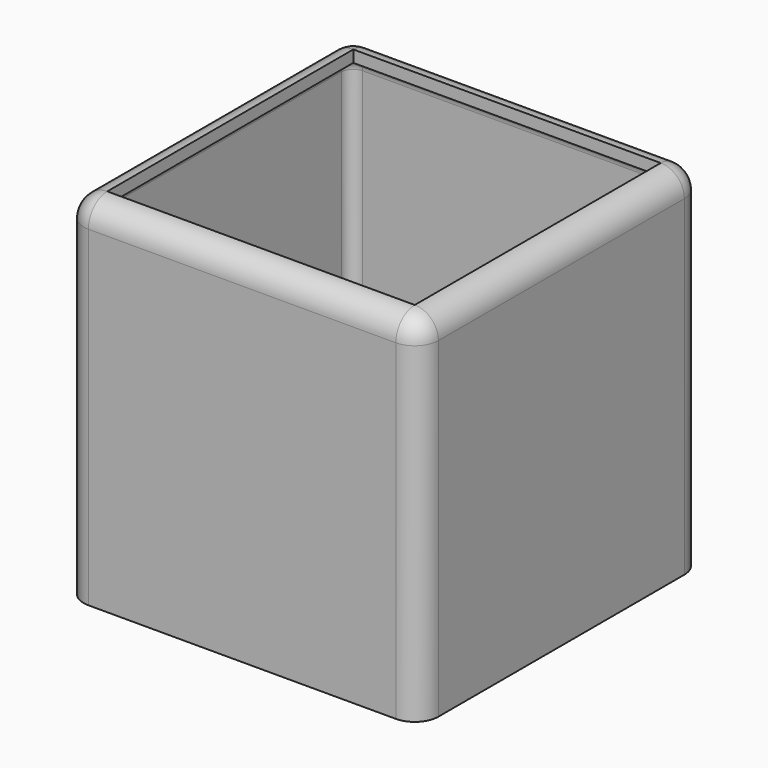
from build123d import *

# Parameters (mm, degrees)
F0_W     = 76.2
F0_H     = 76.2
F1_DEPTH = 76.2
F2_R     = 5.08
F3_T     = -2.54


# Not quite as in the source:
# - a shell that OpenCascade refuses in one call is made with other operations: the cavity is built on its own and cut out


with BuildPart() as f1:
    # F0 (on Top) → F1 (new body)
    with BuildSketch(Plane.XY):
        with Locations((7.7656768262, 2.775496821)):
            Rectangle(F0_W, F0_H)
    extrude(amount=F1_DEPTH)

    # F2
    f2_edges = [f1.edges().sort_by_distance(p)[0] for p in [
        (7.765677, -35.324503, 76.2),
        (45.865677, 2.775497, 76.2),
        (7.765677, 40.875497, 76.2),
        (-30.334323, 2.775497, 76.2),
        (45.865677, -35.324503, 38.1),
        (-30.334323, -35.324503, 38.1),
        (45.865677, 40.875497, 38.1),
        (-30.334323, 40.875497, 38.1),
    ]]
    fillet(f2_edges, radius=F2_R)

    # F3: a shell. OpenCascade refuses it in one call, so the cavity is built on its own and cut out:
    # the body offset inwards by the wall thickness, plus a prism from it out through each open face.
    f3_core = offset(f1.part, amount=F3_T, mode=Mode.PRIVATE)
    f3_exits = [f3_core.faces().sort_by_distance(p)[0] for p in [
        (7.765677, 2.775497, 73.66),
    ]]
    add(f3_core, mode=Mode.SUBTRACT)
    extrude(f3_exits, amount=-F3_T, mode=Mode.SUBTRACT)


solid = f1.part
